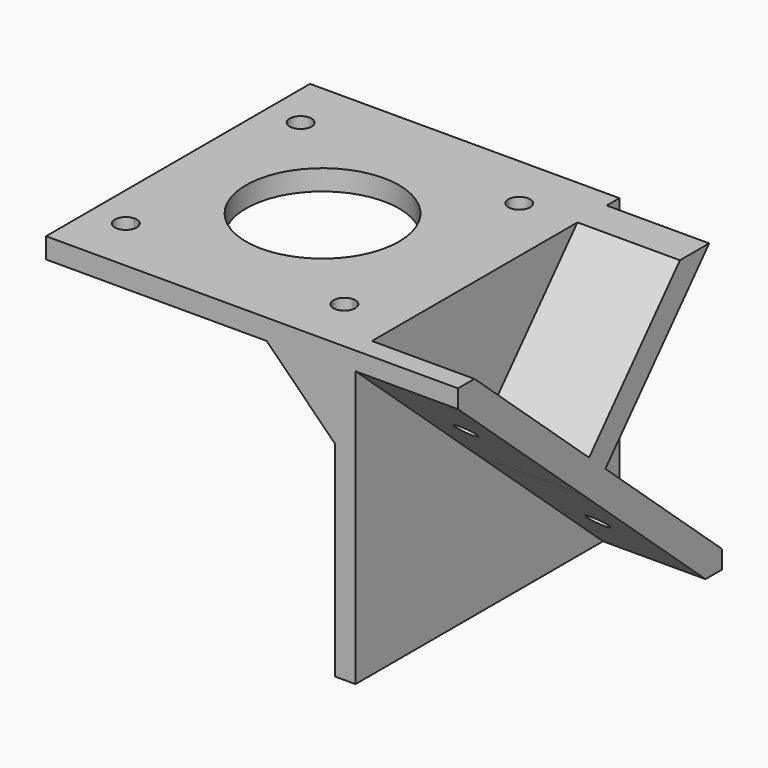
from build123d import *

# Parameters (mm, degrees)
F0_W     = 10
F0_H     = 3
F0_W_2   = 32.3
F0_R     = 11.2
F1_DEPTH = 3
F2_DEPTH = 40
F4_DEPTH = 15
F5_DEPTH = 10
F6_SIZE  = 9.99999
F7_R     = 1.6
F8_R     = 1.6
F9_DEPTH = 25


# Not quite as in the source:
# - a fillet or chamfer is up to 0.001 mm smaller than in the source, because OpenCascade refuses the exact size


with BuildPart() as f1:
    # F0 (on Top) → F1 (new body)
    with BuildSketch(Plane.XY):
        Polygon((21.15, -21.15), (21.15, 21.15), (11.15, 21.15), (-21.15, 21.15), (-21.15, -21.15), (11.15, -21.15), align=None)
        with BuildLine():
            ThreePointArc((-16, 14.4), (-17.1313708499, 17.1313708499), (-14.4, 16))
            Line((-14.4, 16), (14.4, 16))
            ThreePointArc((14.4, 16), (16, 17.6), (17.6, 16))
            ThreePointArc((17.6, 16), (17.1313708499, 14.8686291501), (16, 14.4))
            Line((16, 14.4), (16, -14.4))
            ThreePointArc((16, -14.4), (17.1313708499, -14.8686291501), (17.6, -16))
            ThreePointArc((17.6, -16), (16, -17.6), (14.4, -16))
            Line((14.4, -16), (-14.4, -16))
            ThreePointArc((-14.4, -16), (-17.1313708499, -17.1313708499), (-16, -14.4))
            Line((-16, -14.4), (-16, 14.4))
        make_face(mode=Mode.SUBTRACT)
        Polygon((21.15, 24.15), (21.15, 21.15), (21.15, -21.15), (21.15, -24.15), (24.15, -24.15), (24.15, 24.15), align=None)
        with Locations((16.15, 22.65)):
            Rectangle(F0_W, F0_H)
        with Locations((-5, 22.65)):
            Rectangle(F0_W_2, F0_H)
        with Locations((16.15, -22.65)):
            Rectangle(F0_W, F0_H)
        Polygon((11.15, -24.15), (11.15, -21.15), (-21.15, -21.15), (-21.15, -24.15), (9.2402426526, -24.15), align=None)
        with BuildLine():
            Line((14.4, 16), (-14.4, 16))
            ThreePointArc((-14.4, 16), (-14.8686291501, 14.8686291501), (-16, 14.4))
            Line((-16, 14.4), (-16, -14.4))
            ThreePointArc((-16, -14.4), (-14.8686291501, -14.8686291501), (-14.4, -16))
            Line((-14.4, -16), (14.4, -16))
            ThreePointArc((14.4, -16), (14.8686291501, -14.8686291501), (16, -14.4))
            Line((16, -14.4), (16, 14.4))
            ThreePointArc((16, 14.4), (14.8686291501, 14.8686291501), (14.4, 16))
        make_face()
        Circle(F0_R, mode=Mode.SUBTRACT)
    extrude(amount=F1_DEPTH)

    # F0 (on Top) → F2 (join)
    with BuildSketch(Plane.XY):
        Polygon((21.15, 24.15), (21.15, 21.15), (21.15, -21.15), (21.15, -24.15), (24.15, -24.15), (24.15, 24.15), align=None)
    extrude(amount=-F2_DEPTH)

    # F3 (on face) → F4 (join)
    with BuildSketch(Plane.YZ.offset(24.15)):
        Polygon((-0.1639153264, -15.6763265476), (1.329879063, -17.0062056106), (19.1407867495, 3), (16.4630420556, 3), align=None)
        Polygon((19.1407867495, 3), (1.329879063, -17.0062056106), (2.8236734524, -18.3360846736), (21.8185314434, 3), align=None)
        Polygon((1.329879063, -17.0062056106), (0, -18.5), (24.15, -40), (24.15, -37.3222553061), (2.8236734524, -18.3360846736), align=None)
        Polygon((24.15, -40), (0, -18.5), (-1.329879063, -19.9937943894), (21.1422077043, -40), align=None)
        Polygon((0, -18.5), (-24.15, 3), (-24.15, 0.3222553061), (-1.329879063, -19.9937943894), align=None)
        Polygon((-21.1422077043, 3), (-24.15, 3), (0, -18.5), (1.329879063, -17.0062056106), (-0.1639153264, -15.6763265476), align=None)
    extrude(amount=F4_DEPTH)

    # F0 (on Top) → F5 (join)
    with BuildSketch(Plane.XY):
        with Locations((16.15, 22.65)):
            Rectangle(F0_W, F0_H)
        with Locations((16.15, -22.65)):
            Rectangle(F0_W, F0_H)
    extrude(amount=-F5_DEPTH)

    # F6 (size 10 in the source; OpenCascade refuses exactly that, so slightly less here)
    f6_edges = [f1.edges().sort_by_distance(p)[0] for p in [
        (11.15, 22.65, -10),
        (11.15, -22.65, -10),
    ]]
    chamfer(f6_edges, length=F6_SIZE)

    # F7 (on face) + F8 (on face) → F9 (cut)
    with BuildSketch(Plane(origin=(0, -7.8579881454, -8.8265308702), x_dir=(1, 0, 0), z_dir=(0, 0.6649395315, 0.7468971947))):
        with Locations((31.65, 28.5779957713)):
            Circle(F7_R)
    with BuildSketch(Plane(origin=(0, -7.8579881454, -8.8265308702), x_dir=(1, 0, 0), z_dir=(0, 0.6649395315, 0.7468971947))):
        with Locations((31.65, -3.7422464428)):
            Circle(F8_R)
    extrude(amount=-F9_DEPTH, mode=Mode.SUBTRACT)


solid = f1.part
